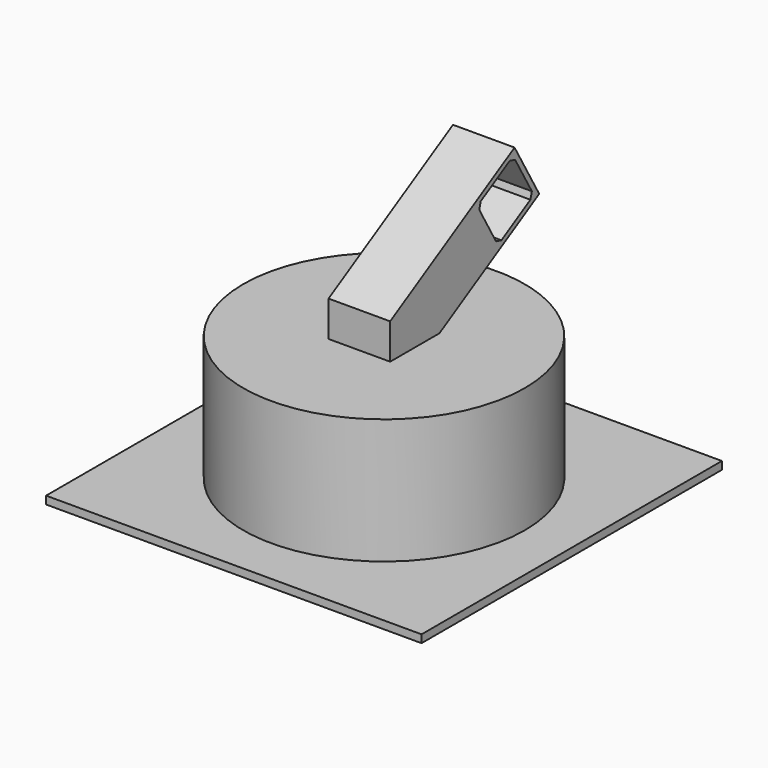
from build123d import *

# Parameters (mm, degrees)
F0_W         = 304.8
F0_H         = 304.8
F1_DEPTH     = 6.35
F2_R         = 114.3
F3_DEPTH     = 101.6
F4_W         = 50
F4_H         = 50
F5_DEPTH     = 28.868
F7_DEPTH     = 50
F9_DEPTH     = 48
F11_DEPTH    = 48
F12_R        = 11
F13_DEPTH    = 9
F15_DEPTH    = 15
F16_T2_ANGLE = 343.7894292622


# Not quite as in the source:
# - a fillet or chamfer that OpenCascade refuses, or shapes differently, is made with other operations: its cross-section is extruded or revolved along the edge and cut away or added


with BuildPart() as f1:
    # F0 (on Top) → F1 (new body)
    with BuildSketch(Plane.XY):
        Rectangle(F0_W, F0_H)
    extrude(amount=F1_DEPTH)

    # F2 (on face) → F3 (join)
    with BuildSketch(Plane.XY.offset(6.35)):
        Circle(F2_R)
    extrude(amount=F3_DEPTH)

    # F10 (on face) → F11 (cut)
    with BuildSketch(Plane.XY.offset(107.95)):
        Polygon((-21.0001030612, 17), (-21.0001030612, -17), (-17, -21.0001030612), (17, -21.0001030612), (21.0001030612, -17), (21.0001030612, 17), (17, 21.0001030612), (-17, 21.0001030612), align=None)
    extrude(amount=-F11_DEPTH, mode=Mode.SUBTRACT)


with BuildPart() as f5:
    # F4 (on face) → F5 (new body)
    with BuildSketch(Plane.XY.offset(107.95)):
        Rectangle(F4_W, F4_H)
    extrude(amount=F5_DEPTH)

    # F6 (on face) → F7 (join)
    with BuildSketch(Plane(origin=(-25, 0, 0), x_dir=(0, -1, 0), z_dir=(-1, 0, 0))):
        Polygon((-25, 136.818), (25, 136.818), (-101.2399952248, 209.7026952255), (-126.2399952248, 166.4014250363), (-25, 107.9504865405), align=None)
    extrude(amount=-F7_DEPTH)

    # F8 (on face) → F9 (cut)
    with BuildSketch(Plane.YZ.offset(25)):
        Polygon((96.3117404639, 202.238682864), (66.8668767352, 185.238682864), (65.4027373971, 179.7744404647), (82.4027373971, 150.329576736), (87.8669797964, 148.8654373978), (117.3118435251, 165.8654373978), (118.7759828632, 171.3296797972), (101.7759828632, 200.7745435258), align=None)
    extrude(amount=-F9_DEPTH, mode=Mode.SUBTRACT)

    # F12 (on face) → F13 (cut)
    with BuildSketch(Plane(origin=(0, 0, 107.95), x_dir=(1, 0, 0), z_dir=(0, 0, -1))):
        Circle(F12_R)
    extrude(amount=-F13_DEPTH, mode=Mode.SUBTRACT)

    # F14 (on face) → F15 (cut)
    with BuildSketch(Plane(origin=(0, 0, 116.95), x_dir=(1, 0, 0), z_dir=(0, 0, -1))):
        with BuildLine():
            Line((1.5, 2), (-1.5, 2))
            ThreePointArc((-1.5, 2), (0, -2.5), (1.5, 2))
        make_face()
    extrude(amount=-F15_DEPTH, mode=Mode.SUBTRACT)

    # F16: fillet of radius 0.5 on 1 edges, made by hand

    # F16_s1 → F16_t2 (revolve)
    with BuildSketch(Plane(origin=(0, 0, 0), x_dir=(0, 0, 1), z_dir=(0.9900106558, -0.1409925581, 0))):
        with BuildLine():
            ThreePointArc((131.45, 2.5), (131.8035533906, 2.3535533906), (131.95, 2))
            Line((131.95, 2), (131.95, 2.5))
            Line((131.95, 2.5), (131.45, 2.5))
        make_face()
    revolve(axis=Axis((0, 0, 131.95), (0, 0, -1)), revolution_arc=F16_T2_ANGLE)


solid = Compound([f1.part, f5.part])
